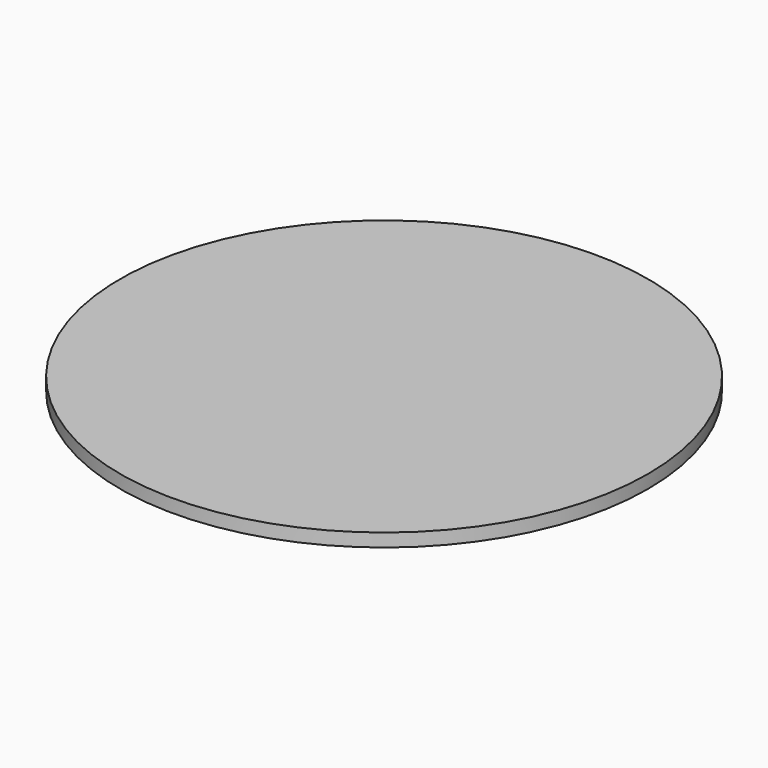
from build123d import *

# Parameters (mm, degrees)
F0_R     = 25.4
F4_DEPTH = 1.27


# Not quite as in the source:
# - the program builds the solid bodies; features that only make, move or delete a surface that nothing else refers to are left out


with BuildPart() as f4:
    # F0 (on Top) → F4 (new body)
    with BuildSketch(Plane.XY):
        Circle(F0_R)
    extrude(amount=-F4_DEPTH)


solid = f4.part
